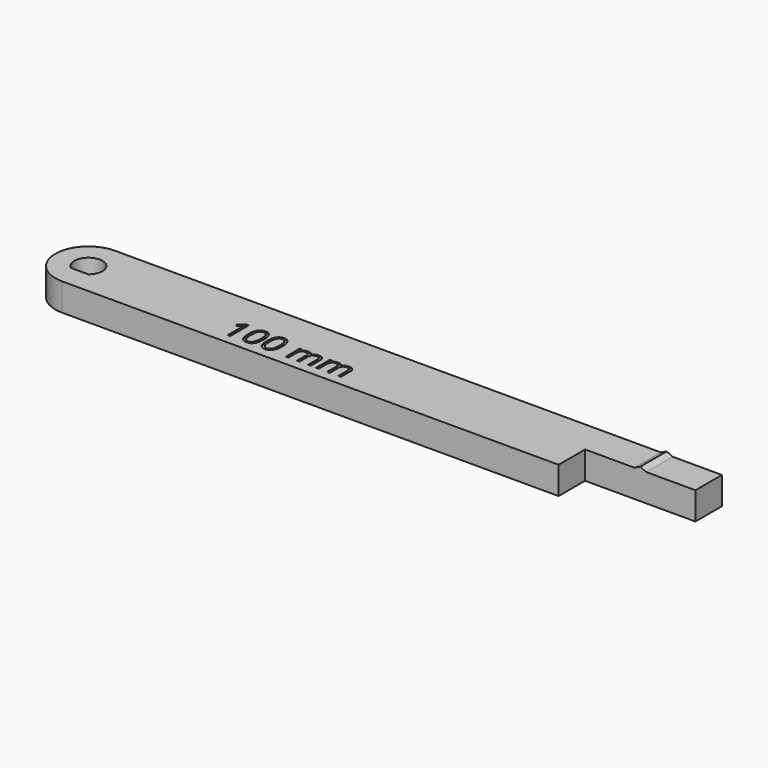
from build123d import *

# Parameters (mm, degrees)
F1_DEPTH     = 5
F3_DEPTH     = 6
F4_TEXT_SIZE = 5.8870730249
F5_DEPTH     = 0.2


# Not quite as in the source:
# - Text() gives the source's letters only with a copy of the font that has no kerning and outlines rounded to 1/6400 em; it was checked with that copy


with BuildPart() as f1:
    # F0 (on Top) → F1 (new body)
    with BuildSketch(Plane.XY):
        with BuildLine():
            ThreePointArc((0, 6), (-6, 0), (0, -6))
            Line((0, -6), (90, -6))
            Line((90, -6), (90, 0))
            Line((90, 0), (110, 0))
            Line((110, 0), (110, 6))
            Line((110, 6), (0, 6))
        make_face()
        with BuildLine():
            ThreePointArc((-1.581929202, -2), (0, 2.55), (1.581929202, -2))
            Line((1.581929202, -2), (-1.581929202, -2))
        make_face(mode=Mode.SUBTRACT)
    extrude(amount=F1_DEPTH)

    # F2 (on face) → F3 (join)
    with BuildSketch(Plane.XZ):
        Polygon((100, 5.5), (98.9277465397, 5), (101.0722534603, 5), align=None)
    extrude(amount=-F3_DEPTH)

    # F4 (on face) → F5 (cut)
    with BuildSketch(Plane.XY.offset(5)):
        with Locations((27.0271468908, -4.2386925779)):
            Text('100 mm', F4_TEXT_SIZE, font='Open Sans', text_align=(TextAlign.LEFT, TextAlign.BOTTOM))
    extrude(amount=-F5_DEPTH, mode=Mode.SUBTRACT)


solid = f1.part
